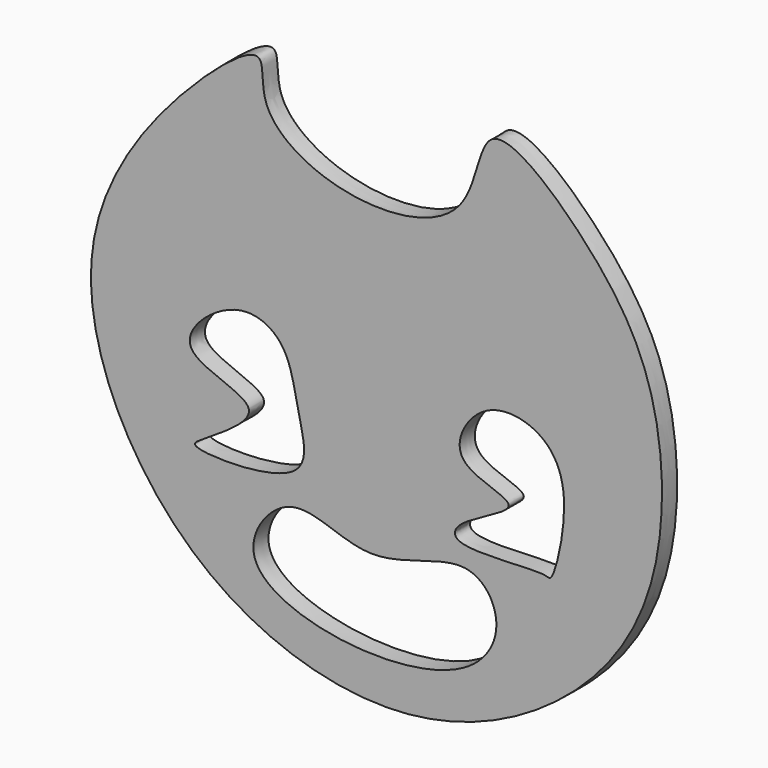
from build123d import *

# Parameters (mm, degrees)
F1_DEPTH = 2
F3_DEPTH = 25
F5_DEPTH = 25


with BuildPart() as f1:
    # F0 (on Front) → F1 (new body)
    with BuildSketch(Plane.XZ):
        with BuildLine():
            add(Edge.make_bspline(
                [(-49.5490767062, 64.0834718943), (-48.9333312885, 63.6575441472), (-50.0473862178, 58.7809579383), (-40.2422780137, 53.0590758533), (-26.2817009426, 55.0093394079), (-26.4039242659, 68.7789394166), (-13.0096656682, 57.1222193065), (-6.619772984, 45.9980926586), (-6.4893058259, 27.9555878027), (-15.8163885409, 14.2275782627), (-34.5537634201, 5.1462980778), (-58.9775502984, 13.1224064881), (-71.9540800422, 39.560792077), (-58.8480202683, 58.0080222816), (-50.4725735578, 64.7222796258), (-49.5490767062, 64.0834718943)],
                knots=[0, 0, 0, 0, 0.0411493462, 0.1069503048, 0.1785591524, 0.2361532995, 0.3075442624, 0.3846516064, 0.4681651457, 0.5495985589, 0.6392533937, 0.7386182864, 0.8420592326, 0.9382840853, 1, 1, 1, 1], degree=3))
        make_face()
    extrude(amount=F1_DEPTH)

    # F2 (on face) → F3 (cut)
    with BuildSketch(Plane.XZ.offset(2)):
        with BuildLine():
            add(Edge.make_bspline(
                [(-50.6061278284, 31.0507565737), (-50.9817318008, 32.4523710945), (-60.5091609085, 33.6656193572), (-52.080496768, 41.3796065461), (-46.2595379356, 38.658936112), (-45.6051769481, 32.5563263033), (-43.1176107758, 25.0825366979), (-57.2786539215, 25.188504599), (-55.539875681, 26.7850853614), (-50.2406390649, 29.686888256), (-50.6061278284, 31.0507565737)],
                knots=[0, 0, 0, 0, 0.1390810183, 0.274416513, 0.3940578073, 0.5228427745, 0.6459471144, 0.8137702355, 0.8646645053, 1, 1, 1, 1], degree=3))
        make_face()
        with BuildLine():
            add(Edge.make_bspline(
                [(-23.1229029596, 31.0507565737), (-23.237129146, 31.867415549), (-30.2625934836, 32.657882679), (-26.4280565006, 40.0208377866), (-19.9168801679, 39.6751090741), (-16.1324990648, 34.6636485349), (-18.3957880768, 25.0747909123), (-19.3534554956, 26.2006993496), (-29.3896150536, 24.9187769805), (-28.5969635462, 28.169318267), (-23.0021234573, 30.187244732), (-23.1229029596, 31.0507565737)],
                knots=[0, 0, 0, 0, 0.1169659491, 0.2329541817, 0.3511422269, 0.4733337166, 0.617773623, 0.6624192019, 0.8127511672, 0.876323551, 1, 1, 1, 1], degree=3))
        make_face()
    extrude(amount=-F3_DEPTH, mode=Mode.SUBTRACT)

    # F4 (on face) → F5 (cut)
    with BuildSketch(Plane.XZ.offset(2)):
        with BuildLine():
            add(Edge.make_bspline(
                [(-46.1136773229, 23.3871657401), (-43.5906896615, 24.0367826301), (-37.8301040064, 19.5288784443), (-27.5048976955, 25.7473622192), (-23.3189967208, 19.8293624238), (-26.8355548191, 12.9651489321), (-41.0011831332, 11.5010443796), (-52.9238132902, 16.5999853568), (-48.3599224178, 22.8088043097), (-46.1136773229, 23.3871657401)],
                knots=[0, 0, 0, 0, 0.1442488127, 0.3013938291, 0.4099502193, 0.5307302503, 0.7155725087, 0.8715736137, 1, 1, 1, 1], degree=3))
        make_face()
    extrude(amount=-F5_DEPTH, mode=Mode.SUBTRACT)


solid = f1.part
